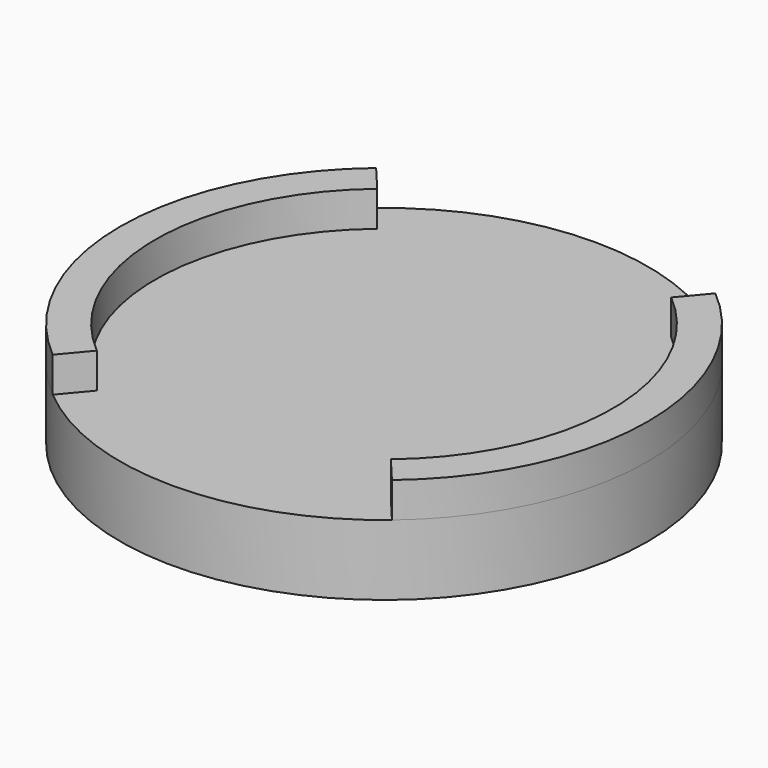
from build123d import *

# Parameters (mm, degrees)
F0_R     = 19.05
F1_DEPTH = 5.08
F3_DEPTH = 2.54


# Not quite as in the source:
# - a pattern or mirror of a feature is missing from the dataset's text; its kind, count and spacing are read off the source's solid


with BuildPart() as f1:
    # F0 (on Top) → F1 (new body)
    with BuildSketch(Plane.XY):
        Circle(F0_R)
    extrude(amount=F1_DEPTH)

    # F2 (on face) → F3 (join)
    with BuildSketch(Plane.XY.offset(5.08)):
        with BuildLine():
            ThreePointArc((-10.6124234359, -12.6473937559), (-16.51, 0), (-10.6124234359, 12.6473937559))
            Line((-10.6124234359, 12.6473937559), (-12.2451039645, 14.5931466414))
            ThreePointArc((-12.2451039645, 14.5931466414), (-19.05, 0), (-12.2451039645, -14.5931466414))
            Line((-12.2451039645, -14.5931466414), (-10.6124234359, -12.6473937559))
        make_face()
    f3 = extrude(amount=F3_DEPTH)

    # F3_copies: F3 across plane
    add(f3.mirror(Plane(origin=(0, 0, 0), x_dir=(0, 0, 1), z_dir=(1, 0, 0))))


solid = f1.part
